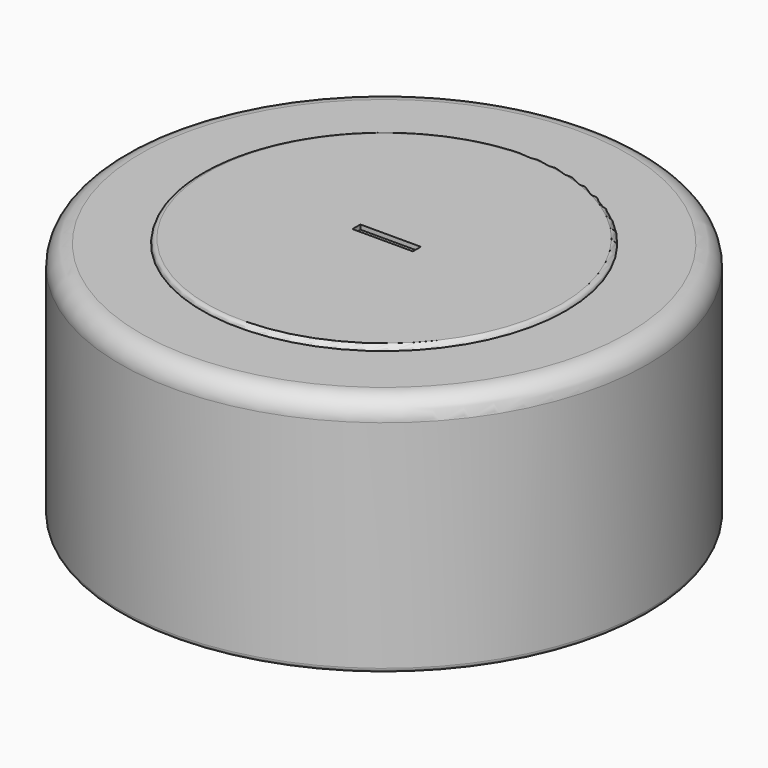
from build123d import *

# Parameters (mm, degrees)
F0_R         = 5.8
F1_DEPTH     = 5.3
F2_R         = 4
F3_DEPTH     = 0.1
F4_R         = 0.09999
F5_R         = 0.45
F6_R         = 0.1
F7_TEXT_SIZE = 3.1974606423
F8_DEPTH     = 0.1
F9_TEXT_SIZE = 2.2743770404
F10_DEPTH    = 0.1


# Not quite as in the source:
# - a fillet or chamfer is up to 0.001 mm smaller than in the source, because OpenCascade refuses the exact size
# - Text() gives the source's letters only with a copy of the font that has no kerning and outlines rounded to 1/6400 em; it was checked with that copy


with BuildPart() as f1:
    # F0 (on Top) → F1 (new body)
    with BuildSketch(Plane.XY):
        Circle(F0_R)
    extrude(amount=F1_DEPTH)

    # F2 (on face) → F3 (join)
    with BuildSketch(Plane.XY.offset(5.3)):
        Circle(F2_R)
    extrude(amount=F3_DEPTH)

    # F4 (radius 0.1 in the source; OpenCascade refuses exactly that, so slightly less here)
    f4_edges = [f1.edges().sort_by_distance(p)[0] for p in [
        (-4, 0, 5.4),
    ]]
    fillet(f4_edges, radius=F4_R)

    # F5
    f5_edges = [f1.edges().sort_by_distance(p)[0] for p in [
        (-5.8, 0, 5.3),
    ]]
    fillet(f5_edges, radius=F5_R)

    # F6
    f6_edges = [f1.edges().sort_by_distance(p)[0] for p in [
        (-5.8, 0, 0),
    ]]
    fillet(f6_edges, radius=F6_R)

    # F7 (on face) → F8 (cut)
    with BuildSketch(Plane.XY.offset(5.4)):
        with Locations((-0.6319797699, 0.4342252796)):
            Text('_', F7_TEXT_SIZE, font='Open Sans', font_style=FontStyle.BOLD, text_align=(TextAlign.LEFT, TextAlign.BOTTOM))
    extrude(amount=-F8_DEPTH, mode=Mode.SUBTRACT)

    # F9 (on face) → F10 (cut)
    with BuildSketch(Plane(origin=(0, 0, 0), x_dir=(1, 0, 0), z_dir=(0, 0, -1))):
        with Locations((-2.7473763905, 2.2979513742)):
            Text('LR44', F9_TEXT_SIZE, font='Open Sans', font_style=FontStyle.BOLD, text_align=(TextAlign.LEFT, TextAlign.BOTTOM))
        with Locations((-0.9744284133, -0.7952014008)):
            Text('+', F9_TEXT_SIZE, font='Open Sans', font_style=FontStyle.BOLD, text_align=(TextAlign.LEFT, TextAlign.BOTTOM))
        with Locations((-2.7473763905, -3.8883541757)):
            Text('1.5V', F9_TEXT_SIZE, font='Open Sans', font_style=FontStyle.BOLD, text_align=(TextAlign.LEFT, TextAlign.BOTTOM))
    extrude(amount=-F10_DEPTH, mode=Mode.SUBTRACT)


solid = f1.part
